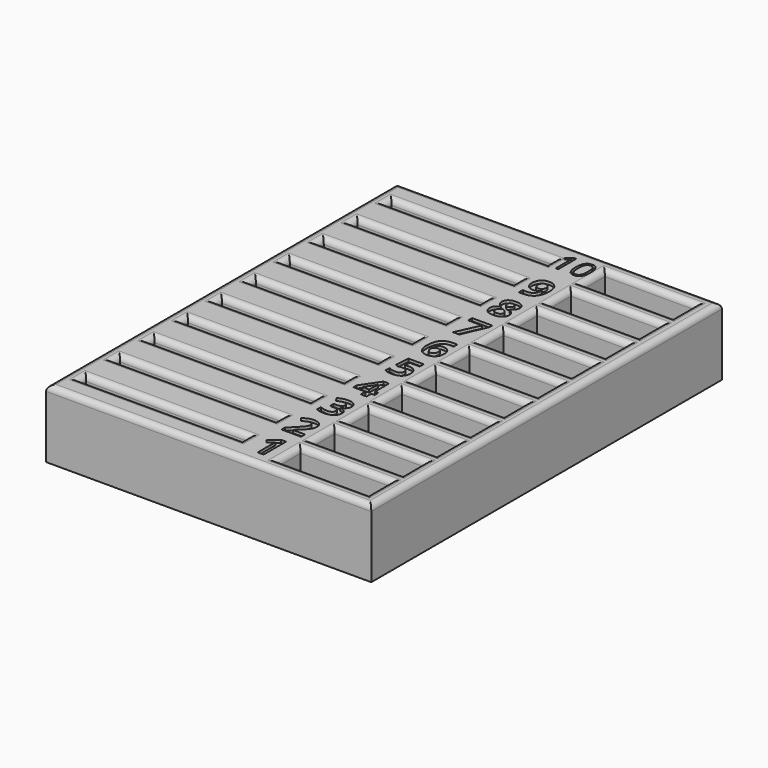
from build123d import *

# Parameters (mm, degrees)
F0_W           = 115
F0_H           = 155
F1_DEPTH       = 24
F2_W           = 32
F2_H           = 10
F2_W_2         = 57.5
F2_H_2         = 3
F3_DEPTH       = 23
F4_R           = 2
F2_TEXT_SIZE   = 13.8888888889
F2_TEXT_SIZE_2 = 11.1111111111
F5_DEPTH       = 1


# Not quite as in the source:
# - a feature names something its author has since deleted; it is built from what else it names
# - Text() gives the source's letters only with a copy of the font that has no kerning and outlines rounded to 1/6400 em; it was checked with that copy


with BuildPart() as f1:
    # F0 (on Top) → F1 (new body)
    with BuildSketch(Plane.XY):
        with Locations((7.6503974199, 49.134781265)):
            Rectangle(F0_W, F0_H)
    extrude(amount=F1_DEPTH)

    # F2 (on face) → F3 (cut)
    with BuildSketch(Plane.XY.offset(24)):
        with Locations((44.1503974199, -18.365218735)):
            Rectangle(F2_W, F2_H)
        with Locations((-16.0996025801, -18.365218735)):
            Rectangle(F2_W_2, F2_H_2)
        with Locations((-16.11783728, -3.365218735)):
            Rectangle(F2_W_2, F2_H_2)
        with Locations((44.2294590175, -3.365218735)):
            Rectangle(F2_W, F2_H)
        with Locations((44.237555936, 11.634781265)):
            Rectangle(F2_W, F2_H)
        with Locations((44.0956111997, 26.634781265)):
            Rectangle(F2_W, F2_H)
        with Locations((43.9957920462, 41.634781265)):
            Rectangle(F2_W, F2_H)
        with Locations((43.9284516543, 56.634781265)):
            Rectangle(F2_W, F2_H)
        with Locations((43.9118291706, 71.634781265)):
            Rectangle(F2_W, F2_H)
        with Locations((43.8242364198, 86.634781265)):
            Rectangle(F2_W, F2_H)
        with Locations((43.7823194534, 101.634781265)):
            Rectangle(F2_W, F2_H)
        with Locations((43.7629665703, 116.634781265)):
            Rectangle(F2_W, F2_H)
        with Locations((-15.9132478945, 11.634781265)):
            Rectangle(F2_W_2, F2_H_2)
        with Locations((-16.0996025801, 26.634781265)):
            Rectangle(F2_W_2, F2_H_2)
        with Locations((-16.0996025801, 41.634781265)):
            Rectangle(F2_W_2, F2_H_2)
        with Locations((-16.0996025801, 56.634781265)):
            Rectangle(F2_W_2, F2_H_2)
        with Locations((-16.0996025801, 71.634781265)):
            Rectangle(F2_W_2, F2_H_2)
        with Locations((-16.0996025801, 86.634781265)):
            Rectangle(F2_W_2, F2_H_2)
        with Locations((-16.0996025801, 101.634781265)):
            Rectangle(F2_W_2, F2_H_2)
        with Locations((-16.0996025801, 116.634781265)):
            Rectangle(F2_W_2, F2_H_2)
    extrude(amount=-F3_DEPTH, mode=Mode.SUBTRACT)

    # F4
    f4_edges = [f1.edges().sort_by_distance(p)[0] for p in [
        (-16.099603, -19.865219, 24),
        (-16.099603, -16.865219, 24),
        (12.650397, -18.365219, 24),
        (-44.849603, -18.365219, 24),
        (44.150397, -13.365219, 24),
        (44.150397, -23.365219, 24),
        (28.150397, -18.365219, 24),
        (60.150397, -18.365219, 24),
        (-16.117837, -1.865219, 24),
        (-16.117837, -4.865219, 24),
        (-44.867837, -3.365219, 24),
        (12.632163, -3.365219, 24),
        (28.229459, -3.365219, 24),
        (44.229459, 1.634781, 24),
        (60.229459, -3.365219, 24),
        (44.229459, -8.365219, 24),
        (44.237556, 6.634781, 24),
        (28.237556, 11.634781, 24),
        (44.237556, 16.634781, 24),
        (60.237556, 11.634781, 24),
        (44.095611, 21.634781, 24),
        (60.095611, 26.634781, 24),
        (44.095611, 31.634781, 24),
        (28.095611, 26.634781, 24),
        (27.995792, 41.634781, 24),
        (43.995792, 46.634781, 24),
        (65.150397, 49.134781, 24),
        (7.650397, -28.365219, 24),
        (7.650397, 126.634781, 24),
        (-49.849603, 49.134781, 24),
        (12.836752, 11.634781, 24),
        (-15.913248, 13.134781, 24),
        (-44.663248, 11.634781, 24),
        (-15.913248, 10.134781, 24),
        (12.650397, 26.634781, 24),
        (-16.099603, 28.134781, 24),
        (-44.849603, 26.634781, 24),
        (-16.099603, 25.134781, 24),
        (-16.099603, 43.134781, 24),
        (-44.849603, 41.634781, 24),
        (-16.099603, 40.134781, 24),
        (12.650397, 41.634781, 24),
        (43.995792, 36.634781, 24),
        (59.995792, 41.634781, 24),
        (-16.099603, 58.134781, 24),
        (-44.849603, 56.634781, 24),
        (-16.099603, 55.134781, 24),
        (12.650397, 56.634781, 24),
        (-16.099603, 73.134781, 24),
        (-44.849603, 71.634781, 24),
        (-16.099603, 70.134781, 24),
        (12.650397, 71.634781, 24),
        (-16.099603, 88.134781, 24),
        (-44.849603, 86.634781, 24),
        (-16.099603, 85.134781, 24),
        (12.650397, 86.634781, 24),
        (-16.099603, 100.134781, 24),
        (12.650397, 101.634781, 24),
        (-16.099603, 103.134781, 24),
        (-44.849603, 101.634781, 24),
        (12.650397, 116.634781, 24),
        (-16.099603, 118.134781, 24),
        (-44.849603, 116.634781, 24),
        (-16.099603, 115.134781, 24),
        (59.928452, 56.634781, 24),
        (43.928452, 61.634781, 24),
        (27.928452, 56.634781, 24),
        (43.928452, 51.634781, 24),
        (43.911829, 66.634781, 24),
        (59.911829, 71.634781, 24),
        (43.911829, 76.634781, 24),
        (27.911829, 71.634781, 24),
        (59.824236, 86.634781, 24),
        (43.824236, 91.634781, 24),
        (27.824236, 86.634781, 24),
        (43.824236, 81.634781, 24),
        (59.782319, 101.634781, 24),
        (43.782319, 106.634781, 24),
        (27.782319, 101.634781, 24),
        (43.782319, 96.634781, 24),
        (43.762967, 121.634781, 24),
        (27.762967, 116.634781, 24),
        (43.762967, 111.634781, 24),
        (59.762967, 116.634781, 24),
    ]]
    fillet(f4_edges, radius=F4_R)

    # F2 (on face) → F5 (cut)
    with BuildSketch(Plane.XY.offset(24)):
        with Locations((17.3150496557, -23.3167728782)):
            Text('1', F2_TEXT_SIZE, font='Open Sans', font_style=FontStyle.BOLD, text_align=(TextAlign.LEFT, TextAlign.BOTTOM))
        with Locations((16.9844282791, -8.540260829)):
            Text('2', F2_TEXT_SIZE, font='Open Sans', font_style=FontStyle.BOLD, text_align=(TextAlign.LEFT, TextAlign.BOTTOM))
        with Locations((17.1315325424, 6.5467171464)):
            Text('3', F2_TEXT_SIZE, font='Open Sans', font_style=FontStyle.BOLD, text_align=(TextAlign.LEFT, TextAlign.BOTTOM))
        with Locations((17.0247917995, 21.5570514649)):
            Text('4', F2_TEXT_SIZE, font='Open Sans', font_style=FontStyle.BOLD, text_align=(TextAlign.LEFT, TextAlign.BOTTOM))
        with Locations((17.1965332702, 36.5776585042)):
            Text('5', F2_TEXT_SIZE, font='Open Sans', font_style=FontStyle.BOLD, text_align=(TextAlign.LEFT, TextAlign.BOTTOM))
        with Locations((16.9153222814, 51.4915303886)):
            Text('6', F2_TEXT_SIZE, font='Open Sans', font_style=FontStyle.BOLD, text_align=(TextAlign.LEFT, TextAlign.BOTTOM))
        with Locations((16.6382705793, 66.4857046306)):
            Text('7', F2_TEXT_SIZE, font='Open Sans', font_style=FontStyle.BOLD, text_align=(TextAlign.LEFT, TextAlign.BOTTOM))
        with Locations((16.4791615232, 81.5759543329)):
            Text('8', F2_TEXT_SIZE, font='Open Sans', font_style=FontStyle.BOLD, text_align=(TextAlign.LEFT, TextAlign.BOTTOM))
        with Locations((16.3248320594, 96.6079812497)):
            Text('9', F2_TEXT_SIZE, font='Open Sans', font_style=FontStyle.BOLD, text_align=(TextAlign.LEFT, TextAlign.BOTTOM))
        with Locations((13.4427947924, 114.030839324)):
            Text('10', F2_TEXT_SIZE_2, font='Open Sans', text_align=(TextAlign.LEFT, TextAlign.BOTTOM))
    extrude(amount=-F5_DEPTH, mode=Mode.SUBTRACT)


solid = f1.part
